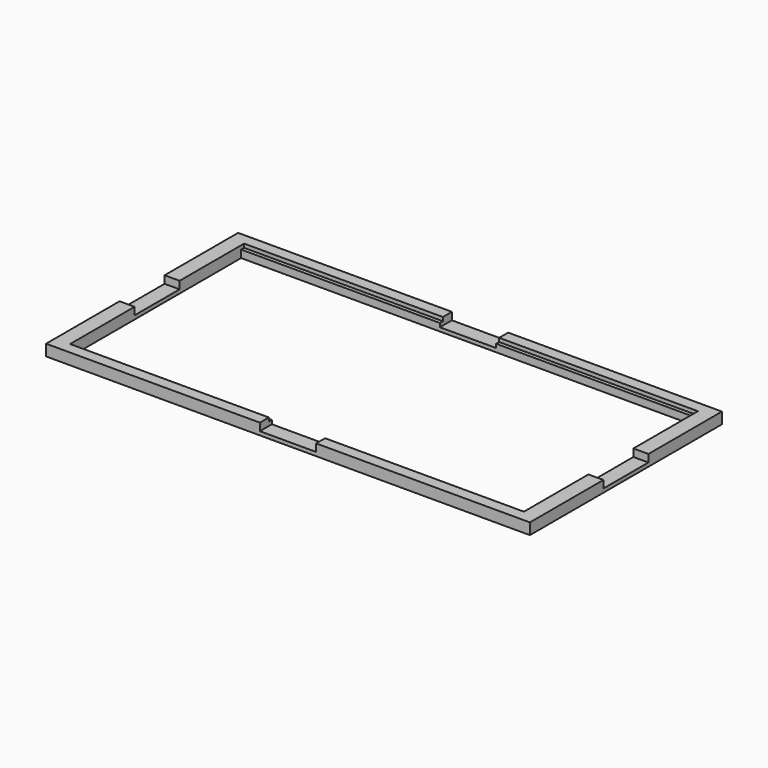
from build123d import *

# Parameters (mm, degrees)
F0_W     = 129
F0_H     = 64
F0_W_2   = 123
F0_H_2   = 58
F0_W_3   = 121
F0_H_3   = 56
F1_DEPTH = 2
F2_W     = 129
F2_H     = 64
F3_DEPTH = 1
F4_W     = 15
F4_H     = 36.0279009569
F4_H_2   = 3
F4_H_3   = 6.1532862581
F4_W_2   = 4
F4_H_4   = 15
F4_W_3   = 3.5279009569
F4_W_4   = 37.6532862581
F5_DEPTH = 2


with BuildPart() as f1:
    # F0 (on Top) → F1 (new body)
    with BuildSketch(Plane.XY):
        with Locations((-61.5, -29)):
            Rectangle(F0_W, F0_H)
        with Locations((-61.5, -29)):
            Rectangle(F0_W_2, F0_H_2, mode=Mode.SUBTRACT)
        with Locations((-61.5, -29)):
            Rectangle(F0_W_2, F0_H_2)
        with Locations((-61.5, -29)):
            Rectangle(F0_W_3, F0_H_3, mode=Mode.SUBTRACT)
    extrude(amount=F1_DEPTH)

    # F2 (on face) → F3 (join)
    with BuildSketch(Plane.XY.offset(2)):
        with Locations((-61.5, -29)):
            Rectangle(F2_W, F2_H)
        Polygon((-122, 0), (-1, 0), (-1, -1), (-1, -57), (-1, -58), (-122, -58), (-122, -57), (-122, -1), align=None, mode=Mode.SUBTRACT)
    extrude(amount=F3_DEPTH)

    # F4 (on face) → F5 (cut)
    with BuildSketch(Plane.XY.offset(3)):
        with Locations((-61.5, 21.0139504785)):
            Rectangle(F4_W, F4_H)
        with Locations((-61.5, 1.5)):
            Rectangle(F4_W, F4_H_2)
        with Locations((-61.5, -3.0766431291)):
            Rectangle(F4_W, F4_H_3)
        with Locations((1, -29)):
            Rectangle(F4_W_2, F4_H_4)
        with Locations((4.7639504785, -29)):
            Rectangle(F4_W_3, F4_H_4)
        with Locations((-19.8266431291, -29)):
            Rectangle(F4_W_4, F4_H_4)
        with Locations((-61.5, -59.5)):
            Rectangle(F4_W, F4_H_2)
        with Locations((-61.5, -54.9233568709)):
            Rectangle(F4_W, F4_H_3)
        with Locations((-61.5, -79.0139504785)):
            Rectangle(F4_W, F4_H)
        with Locations((-103.1733568709, -29)):
            Rectangle(F4_W_4, F4_H_4)
        with Locations((-124, -29)):
            Rectangle(F4_W_2, F4_H_4)
        with Locations((-127.7639504785, -29)):
            Rectangle(F4_W_3, F4_H_4)
    extrude(amount=-F5_DEPTH, mode=Mode.SUBTRACT)


solid = f1.part
